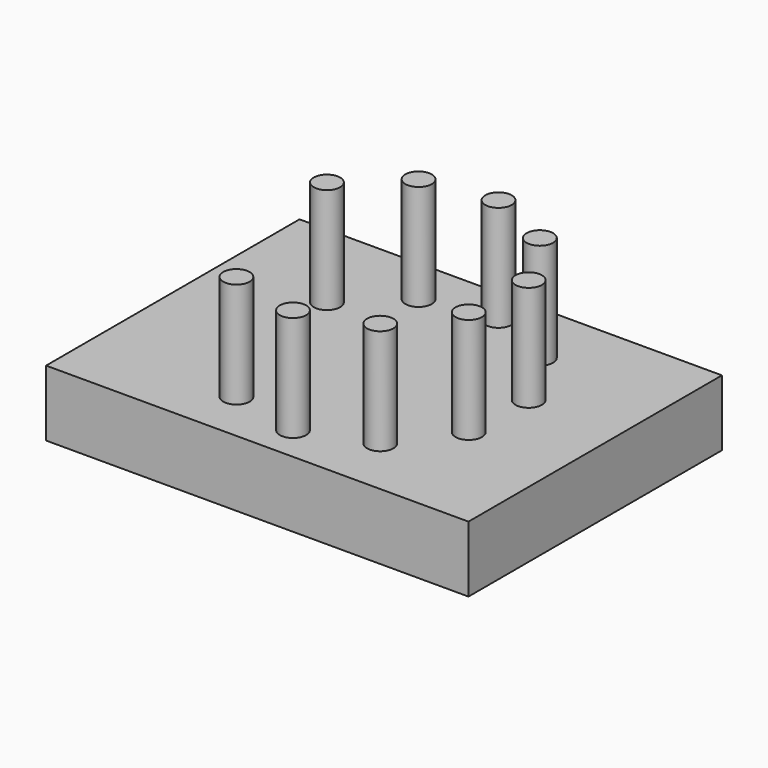
from build123d import *

# Parameters (mm, degrees)
F0_W            = 160
F0_H            = 120
F1_DEPTH        = 25
F2_R            = 5
F4_DEPTH        = 40
F4_COPIES_COUNT = 9
F4_COPIES_ANGLE = 270


# Not quite as in the source:
# - a pattern or mirror of a feature is missing from the dataset's text; its kind, count and spacing are read off the source's solid


with BuildPart() as f1:
    # F0 (on Top) → F1 (new body)
    with BuildSketch(Plane.XY):
        with Locations((-35.207672789, -2.114020288)):
            Rectangle(F0_W, F0_H)
    extrude(amount=F1_DEPTH)

    # F2 (on face) → F4 (join)
    with BuildSketch(Plane.XY.offset(25)):
        with Locations((-75.6510049105, 21.4327722788)):
            Circle(F2_R)
    f4 = extrude(amount=F4_DEPTH)

    # F4_copies: F4 ×9 about axis
    f4_copies_axis = Axis((-35.207673, -2.11402, 0), (0, 0, -1))
    for i in range(1, F4_COPIES_COUNT):
        add(f4.rotate(f4_copies_axis, i * F4_COPIES_ANGLE / (F4_COPIES_COUNT - 1)))


solid = f1.part
